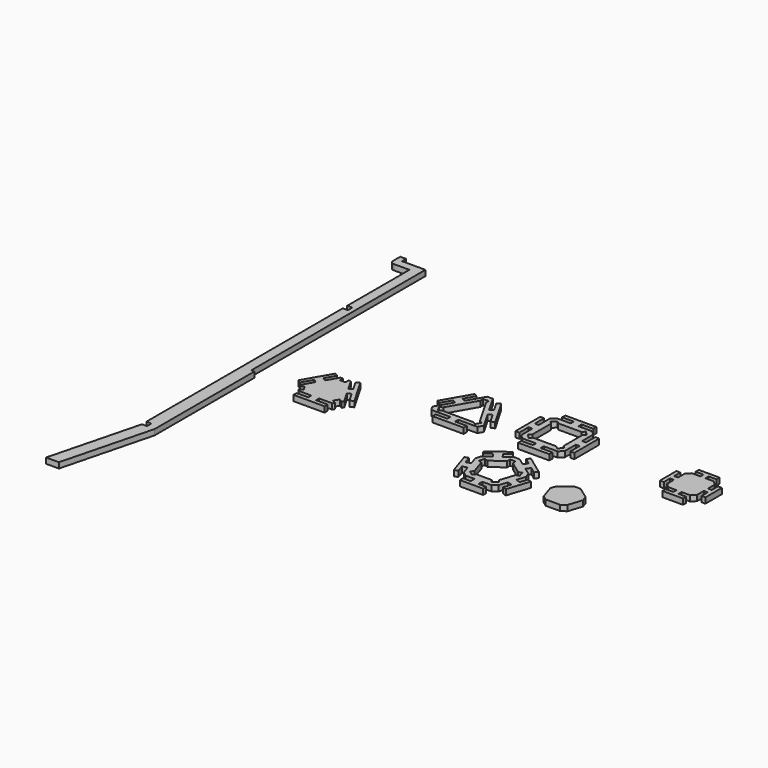
from build123d import *

# Parameters (mm, degrees)
F1_W     = 44.45
F1_H     = 25.4
F2_DEPTH = 18.288
F1_W_2   = 38.1
F1_H_2   = 12.7


# Not quite as in the source:
# - a variable given as a bare number and used for a length is read in inches; the dataset says mm whatever the document's units were


with BuildPart() as f2:
    # F1 (on Top) → F2 (new body)
    with BuildSketch(Plane.XY):
        Polygon((0, 413.512), (0, 0), (31.75, 0), (31.75, 685.8), (0, 685.8), (0, 431.8), (16.51, 431.8), (16.51, 413.512), align=None)
        Polygon((31.75, 0), (0, 0), (0, -388.112), (16.51, -388.112), (16.51, -406.4), (41.91, -406.4), (41.91, 0), align=None)
        Polygon((16.51, -406.4), (0, -406.4), (-76.2, -702.31), (-34.29, -702.31), (41.91, -406.4), align=None)
        with BuildLine():
            Line((-50.8, 685.8), (-44.45, 685.8))
            Line((-44.45, 685.8), (-44.45, 711.2))
            Line((-44.45, 711.2), (-44.45, 727.71))
            Line((-44.45, 727.71), (-63.5, 727.71))
            Line((-63.5, 727.71), (-63.5, 698.5))
            ThreePointArc((-63.5, 698.5), (-59.7802561211, 689.5197438789), (-50.8, 685.8))
        make_face()
        Polygon((0, 685.8), (31.75, 685.8), (31.75, 711.2), (12.7, 711.2), (0, 711.2), align=None)
        with Locations((-22.225, 698.5)):
            Rectangle(F1_W, F1_H)
    extrude(amount=F2_DEPTH)


with BuildPart() as f2b:
    # F1 (on Top) → F2, piece 2 (new body)
    with BuildSketch(Plane.XY):
        Polygon((260.35, 111.6867036526), (260.35, 98.9867036526), (308.356, 15.8378725844), (319.3545226281, 9.4878725844), (323.0206968374, 15.8378725844), (301.7015226281, 52.7637654904), (289.0015226281, 74.7608107465), (267.6823484187, 111.6867036526), align=None)
        Polygon((242.062, 98.9867036526), (194.056, 15.8378725844), (203.2, 0), (299.212, 0), (308.356, 15.8378725844), (260.35, 98.9867036526), align=None)
        Polygon((299.212, 0), (203.2, 0), (192.2014773719, -6.35), (195.8676515813, -12.7), (238.506, -12.7), (263.906, -12.7), (306.5443484187, -12.7), (310.2105226281, -6.35), align=None)
        Polygon((183.0574773719, 9.4878725844), (194.056, 15.8378725844), (242.062, 98.9867036526), (242.062, 111.6867036526), (234.7296515813, 111.6867036526), (213.4104773719, 74.7608107465), (200.7104773719, 52.7637654904), (179.3913031626, 15.8378725844), align=None)
        Polygon((189.7119547439, 59.1137654904), (200.7104773719, 52.7637654904), (213.4104773719, 74.7608107465), (202.4119547439, 81.1108107465), (221.4619547439, 114.1063786307), (210.4634321158, 120.4563786307), (185.0634321158, 76.4622881185), (159.6634321158, 32.4681976062), (170.6619547439, 26.1181976062), align=None)
        Polygon((300.0000452561, 81.1108107465), (289.0015226281, 74.7608107465), (301.7015226281, 52.7637654904), (312.7000452561, 59.1137654904), (331.7500452561, 26.1181976062), (342.7485678842, 32.4681976062), (317.3485678842, 76.4622881185), (291.9485678842, 120.4563786307), (280.9500452561, 114.1063786307), align=None)
        Polygon((263.906, -12.7), (238.506, -12.7), (238.506, -25.4), (200.406, -25.4), (200.406, -38.1), (251.206, -38.1), (302.006, -38.1), (302.006, -25.4), (263.906, -25.4), align=None)
    extrude(amount=F2_DEPTH)


with BuildPart() as f2c:
    # F1 (on Top) → F2, piece 3 (new body)
    with BuildSketch(Plane.XY):
        Polygon((548.6804278352, 186.6284404686), (517.5320529443, 132.6778725844), (526.6760529443, 116.84), (588.9728027261, 116.84), (614.3728027261, 116.84), (676.6695525078, 116.84), (685.8135525078, 132.6778725844), (654.6651776169, 186.6284404686), (641.9651776169, 208.6254857247), (610.8168027261, 262.5760536089), (592.5288027261, 262.5760536089), (561.3804278352, 208.6254857247), align=None)
        Polygon((531.8301323608, 140.9328725844), (541.7288027261, 146.6478725844), (592.5288027261, 234.6360536089), (592.5288027261, 246.0660536089), (610.8168027261, 246.0660536089), (610.8168027261, 234.6360536089), (661.6168027261, 146.6478725844), (671.5154730913, 140.9328725844), (662.3714730913, 125.095), (652.4728027261, 130.81), (550.8728027261, 130.81), (540.9741323608, 125.095), align=None, mode=Mode.SUBTRACT)
        Polygon((652.963700245, 214.9754857247), (641.9651776169, 208.6254857247), (654.6651776169, 186.6284404686), (665.663700245, 192.9784404686), (676.6622228731, 199.3284404686), (670.3122228731, 210.3269630967), (663.9622228731, 221.3254857247), align=None)
        Polygon((537.6819052071, 192.9784404686), (548.6804278352, 186.6284404686), (561.3804278352, 208.6254857247), (550.3819052071, 214.9754857247), (539.3833825791, 221.3254857247), (533.0333825791, 210.3269630967), (526.6833825791, 199.3284404686), align=None)
        Polygon((539.3833825791, 221.3254857247), (550.3819052071, 214.9754857247), (569.4319052071, 247.9710536089), (558.4333825791, 254.3210536089), align=None)
        Polygon((518.6319052071, 159.9828725844), (537.6819052071, 192.9784404686), (526.6833825791, 199.3284404686), (507.6333825791, 166.3328725844), align=None)
        Polygon((633.913700245, 247.9710536089), (652.963700245, 214.9754857247), (663.9622228731, 221.3254857247), (644.9122228731, 254.3210536089), align=None)
        Polygon((676.6622228731, 199.3284404686), (665.663700245, 192.9784404686), (684.713700245, 159.9828725844), (695.7122228731, 166.3328725844), align=None)
        with Locations((633.4228027261, 97.79)):
            Rectangle(F1_W_2, F1_H_2)
        Polygon((614.3728027261, 116.84), (588.9728027261, 116.84), (588.9728027261, 104.14), (588.9728027261, 91.44), (601.6728027261, 91.44), (614.3728027261, 91.44), (614.3728027261, 104.14), align=None)
        with Locations((569.9228027261, 97.79)):
            Rectangle(F1_W_2, F1_H_2)
    extrude(amount=F2_DEPTH)


with BuildPart() as f2d:
    # F1 (on Top) → F2, piece 4 (new body)
    with BuildSketch(Plane.XY):
        Polygon((850.8796180671, 280.514333905), (805.7230546008, 280.514333905), (792.7914857864, 267.5827650906), (792.7914857864, 222.4262016243), (792.7914857864, 197.0262016243), (792.7914857864, 151.8696381579), (805.7230546008, 138.9380693436), (850.8796180671, 138.9380693436), (876.2796180671, 138.9380693436), (921.4361815335, 138.9380693436), (934.3677503478, 151.8696381579), (934.3677503478, 197.0262016243), (934.3677503478, 222.4262016243), (934.3677503478, 267.5827650906), (921.4361815335, 280.514333905), (876.2796180671, 280.514333905), align=None)
        Polygon((817.3973875582, 268.8400009476), (825.4796180671, 260.7577704386), (901.6796180671, 260.7577704386), (909.7618485761, 268.8400009476), (922.6934173904, 255.9084321332), (914.6111868815, 247.8262016243), (914.6111868815, 171.6262016243), (922.6934173904, 163.5439711153), (909.7618485761, 150.612402301), (901.6796180671, 158.6946328099), (825.4796180671, 158.6946328099), (817.3973875582, 150.612402301), (804.4658187438, 163.5439711153), (812.5480492528, 171.6262016243), (812.5480492528, 247.8262016243), (804.4658187438, 255.9084321332), align=None, mode=Mode.SUBTRACT)
        Polygon((850.8796180671, 293.214333905), (850.8796180671, 280.514333905), (876.2796180671, 280.514333905), (876.2796180671, 293.214333905), (914.3796180671, 293.214333905), (914.3796180671, 305.914333905), (863.5796180671, 305.914333905), (812.7796180671, 305.914333905), (812.7796180671, 293.214333905), align=None)
        Polygon((792.7914857864, 197.0262016243), (792.7914857864, 222.4262016243), (780.0914857864, 222.4262016243), (780.0914857864, 260.5262016243), (767.3914857864, 260.5262016243), (767.3914857864, 209.7262016243), (767.3914857864, 158.9262016243), (780.0914857864, 158.9262016243), (780.0914857864, 197.0262016243), align=None)
        Polygon((947.0677503478, 222.4262016243), (934.3677503478, 222.4262016243), (934.3677503478, 197.0262016243), (947.0677503478, 197.0262016243), (947.0677503478, 158.9262016243), (959.7677503478, 158.9262016243), (959.7677503478, 209.7262016243), (959.7677503478, 260.5262016243), (947.0677503478, 260.5262016243), align=None)
        Polygon((876.2796180671, 138.9380693436), (850.8796180671, 138.9380693436), (850.8796180671, 126.2380693436), (812.7796180671, 126.2380693436), (812.7796180671, 113.5380693436), (863.5796180671, 113.5380693436), (914.3796180671, 113.5380693436), (914.3796180671, 126.2380693436), (876.2796180671, 126.2380693436), align=None)
    extrude(amount=F2_DEPTH)


with BuildPart() as f2e:
    # F1 (on Top) → F2, piece 5 (new body)
    with BuildSketch(Plane.XY):
        Polygon((896.2843934283, 27.7588613959), (872.7236180671, 44.8767666886), (854.4356180671, 44.8767666886), (830.8748427059, 27.7588613959), (810.3258110488, 12.8291159877), (786.7650356876, -4.288789305), (781.1137328945, -21.681710875), (790.1131482811, -49.3790634548), (797.9621799383, -73.5358989687), (806.9615953249, -101.2332515485), (821.7568981181, -111.9826682424), (850.8796180671, -111.9826682424), (876.2796180671, -111.9826682424), (905.4023380162, -111.9826682424), (920.1976408093, -101.2332515485), (929.197056196, -73.5358989687), (937.0460878531, -49.3790634548), (946.0455032398, -21.681710875), (940.3942004467, -4.288789305), (916.8334250855, 12.8291159877), align=None)
        Polygon((813.3375547529, -12.9227241278), (854.4356180671, 16.9367666886), (854.4356180671, 28.3667666886), (872.7236180671, 28.3667666886), (872.7236180671, 16.9367666886), (913.8216813814, -12.9227241278), (924.6922573626, -9.3906598821), (930.3435601558, -26.7835814521), (919.4729841745, -30.3156456978), (903.7749208603, -78.6293167256), (910.493306294, -87.8763809713), (895.6980035008, -98.6257976652), (888.9796180671, -89.3787334195), (838.1796180671, -89.3787334195), (831.4612326334, -98.6257976652), (816.6659298403, -87.8763809713), (823.384315274, -78.6293167256), (807.6862519598, -30.3156456978), (796.8156759785, -26.7835814521), (802.4669787716, -9.3906598821), align=None, mode=Mode.SUBTRACT)
        Polygon((876.2796180671, -127.8576682424), (876.2796180671, -111.9826682424), (850.8796180671, -111.9826682424), (850.8796180671, -127.8576682424), (825.4796180671, -127.8576682424), (825.4796180671, -140.5576682424), (863.5796180671, -140.5576682424), (901.6796180671, -140.5576682424), (901.6796180671, -127.8576682424), align=None)
        Polygon((797.9621799383, -73.5358989687), (790.1131482811, -49.3790634548), (775.015126085, -54.2847082405), (767.1660944278, -30.1278727266), (755.0876766709, -34.0523885551), (766.8612241566, -70.287641826), (778.6347716423, -106.5228950968), (790.7131893992, -102.5983792683), (782.8641577421, -78.4415437544), align=None)
        Polygon((810.3258110488, 12.8291159877), (830.8748427059, 27.7588613959), (821.5437518258, 40.6020061816), (842.0927834829, 55.5317515899), (834.6279107788, 65.8062674184), (803.8043632931, 43.4116493061), (772.9808158074, 21.0170311937), (780.4456885115, 10.7425153652), (800.9947201687, 25.6722607734), align=None)
        Polygon((905.6154843085, 40.6020061816), (896.2843934283, 27.7588613959), (916.8334250855, 12.8291159877), (926.1645159656, 25.6722607734), (946.7135476227, 10.7425153652), (954.1784203268, 21.0170311937), (923.3548728412, 43.4116493061), (892.5313253555, 65.8062674184), (885.0664526514, 55.5317515899), align=None)
        Polygon((952.1441100493, -54.2847082405), (937.0460878531, -49.3790634548), (929.197056196, -73.5358989687), (944.2950783922, -78.4415437544), (936.4460467351, -102.5983792683), (948.524464492, -106.5228950968), (960.2980119777, -70.287641826), (972.0715594634, -34.0523885551), (959.9931417064, -30.1278727266), align=None)
    extrude(amount=F2_DEPTH)


with BuildPart() as f2f:
    # F1 (on Top) → F2, piece 6 (new body)
    with BuildSketch(Plane.XY):
        Polygon((1291.8321056824, 258.5733704386), (1264.1715056824, 258.5733704386), (1251.2399368681, 245.6418016243), (1251.2399368681, 217.9812016243), (1251.2399368681, 201.4712016243), (1251.2399368681, 173.8106016243), (1264.1715056824, 160.8790328099), (1291.8321056824, 160.8790328099), (1308.3421056824, 160.8790328099), (1336.0027056824, 160.8790328099), (1348.9342744968, 173.8106016243), (1348.9342744968, 201.4712016243), (1348.9342744968, 217.9812016243), (1348.9342744968, 245.6418016243), (1336.0027056824, 258.5733704386), (1308.3421056824, 258.5733704386), align=None)
        Polygon((1291.8321056824, 271.2733704386), (1291.8321056824, 258.5733704386), (1308.3421056824, 258.5733704386), (1308.3421056824, 271.2733704386), (1333.7421056824, 271.2733704386), (1333.7421056824, 283.9733704386), (1300.0871056824, 283.9733704386), (1266.4321056824, 283.9733704386), (1266.4321056824, 271.2733704386), align=None)
        Polygon((1251.2399368681, 201.4712016243), (1251.2399368681, 217.9812016243), (1238.5399368681, 217.9812016243), (1238.5399368681, 243.3812016243), (1225.8399368681, 243.3812016243), (1225.8399368681, 209.7262016243), (1225.8399368681, 176.0712016243), (1238.5399368681, 176.0712016243), (1238.5399368681, 201.4712016243), align=None)
        Polygon((1308.3421056824, 160.8790328099), (1291.8321056824, 160.8790328099), (1291.8321056824, 148.1790328099), (1266.4321056824, 148.1790328099), (1266.4321056824, 135.4790328099), (1300.0871056824, 135.4790328099), (1333.7421056824, 135.4790328099), (1333.7421056824, 148.1790328099), (1308.3421056824, 148.1790328099), align=None)
        Polygon((1361.6342744968, 217.9812016243), (1348.9342744968, 217.9812016243), (1348.9342744968, 201.4712016243), (1361.6342744968, 201.4712016243), (1361.6342744968, 176.0712016243), (1374.3342744968, 176.0712016243), (1374.3342744968, 209.7262016243), (1374.3342744968, 243.3812016243), (1361.6342744968, 243.3812016243), align=None)
    extrude(amount=F2_DEPTH)


with BuildPart() as f2g:
    # F1 (on Top) → F2, piece 7 (new body)
    with BuildSketch(Plane.XY):
        Polygon((1096.343277984, 14.2766460243), (1077.6507863471, 14.2766460243), (1039.3473913382, -13.5523994167), (1033.5710937552, -31.3300153937), (1048.2016887641, -76.3583567916), (1063.3242321655, -87.3455277044), (1110.6698321655, -87.3455277044), (1125.792375567, -76.3583567916), (1140.4229705759, -31.3300153937), (1134.6466729929, -13.5523994167), align=None)
    extrude(amount=F2_DEPTH)


solid = Compound([f2.part, f2b.part, f2c.part, f2d.part, f2e.part, f2f.part, f2g.part])
